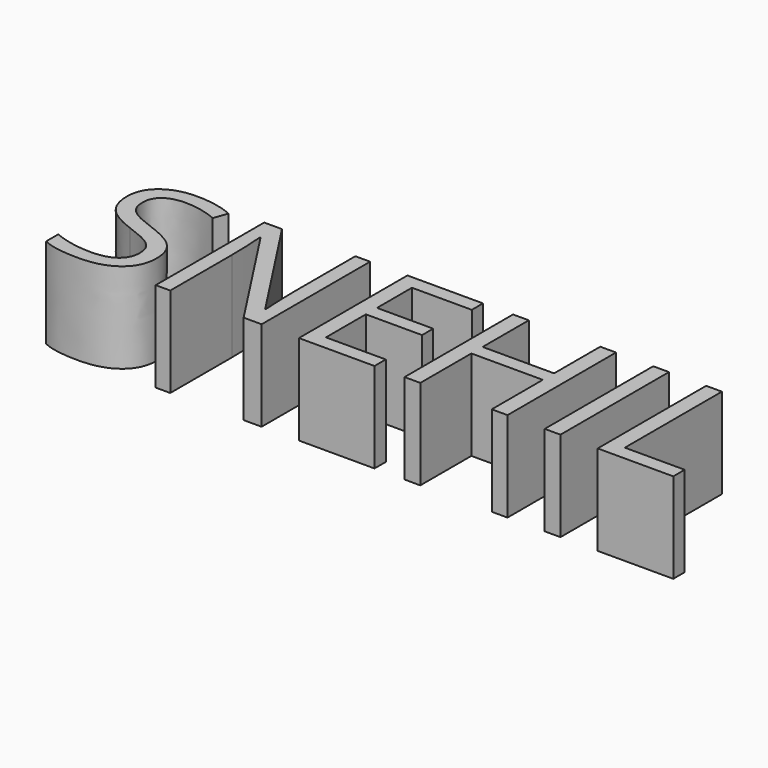
from build123d import *

# Parameters (mm, degrees)
F0_TEXT_SIZE = 26.7423316084
F1_DEPTH     = 12.7


# Not quite as in the source:
# - Text() gives the source's letters only with a copy of the font that has no kerning and outlines rounded to 1/6400 em; it was checked with that copy


with BuildPart() as f1:
    # F0 (on Top) → F1 (new body)
    with BuildSketch(Plane.XY):
        with Locations((-45.9487577394, 31.3522776034)):
            Text('SNEHIL', F0_TEXT_SIZE, font='Open Sans', text_align=(TextAlign.LEFT, TextAlign.BOTTOM))
    extrude(amount=F1_DEPTH)


solid = f1.part
